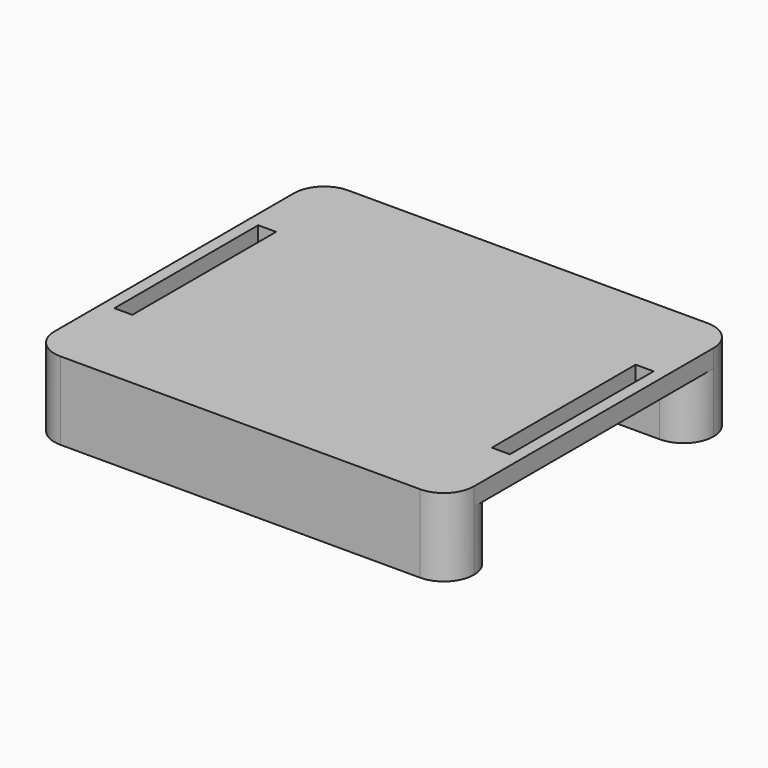
from build123d import *

# Parameters (mm, degrees)
F0_W     = 70
F0_H     = 60
F1_DEPTH = 3
F2_W     = 3
F2_H     = 30
F3_DEPTH = 25
F4_W     = 70
F4_H     = 10
F5_DEPTH = 10
F6_R     = 4.99999


# Not quite as in the source:
# - a fillet or chamfer is up to 0.001 mm smaller than in the source, because OpenCascade refuses the exact size


with BuildPart() as f1:
    # F0 (on Top) → F1 (new body)
    with BuildSketch(Plane.XY):
        Rectangle(F0_W, F0_H)
    extrude(amount=F1_DEPTH)

    # F2 (on Top) → F3 (cut)
    with BuildSketch(Plane.XY):
        with Locations((31.5, 0)):
            Rectangle(F2_W, F2_H)
        with Locations((-31.5, 0)):
            Rectangle(F2_W, F2_H)
    extrude(amount=F3_DEPTH, mode=Mode.SUBTRACT)

    # F4 (on Top) → F5 (join)
    with BuildSketch(Plane.XY):
        with Locations((0, 25)):
            Rectangle(F4_W, F4_H)
        with Locations((0, -25)):
            Rectangle(F4_W, F4_H)
    extrude(amount=-F5_DEPTH)

    # F6 (radius 5 in the source; OpenCascade refuses exactly that, so slightly less here)
    f6_edges = [f1.edges().sort_by_distance(p)[0] for p in [
        (35, -30, -3.5),
        (-35, -30, -3.5),
        (-35, -20, -5),
        (35, -20, -5),
        (35, 20, -5),
        (35, 30, -3.5),
        (-35, 20, -5),
        (-35, 30, -3.5),
    ]]
    fillet(f6_edges, radius=F6_R)


solid = f1.part
